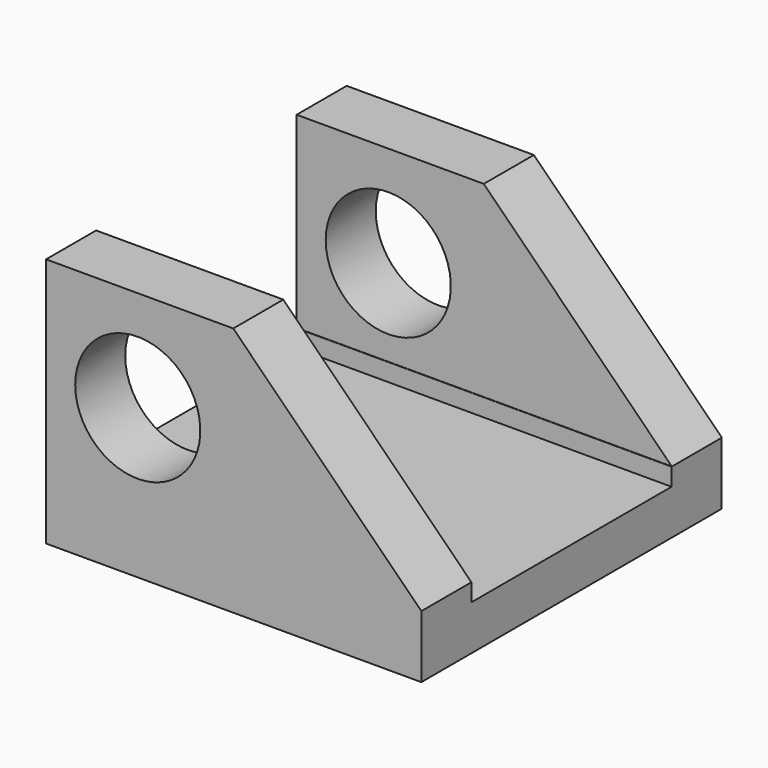
from build123d import *

# Parameters (mm, degrees)
F0_W      = 152.3780375719
F0_H      = 152.3780375719
F1_DEPTH  = 25.4
F3_W      = 76.005205512
F3_H      = 76.2
F4_DEPTH  = 25.4
F6_DEPTH  = 25.4
F9_D      = 50.8
F10_W     = 101.6018704236
F10_H     = 7.1799890138
F11_DEPTH = 152.4


with BuildPart() as f1:
    # F0 (on Top) → F1 (new body)
    with BuildSketch(Plane.XY):
        with Locations((0.1838132739, -0.0919029117)):
            Rectangle(F0_W, F0_H)
    extrude(amount=-F1_DEPTH)



with BuildPart() as f4:
    # F3 (on face) → F4 (new body)
    with BuildSketch(Plane.XZ.offset(76.2809216976)):
        with Locations((-38.002602756, 38.1)):
            Rectangle(F3_W, F3_H)
    extrude(amount=-F4_DEPTH)


with BuildPart() as f6:
    # F5 (on face) → F6 (new body)
    with BuildSketch(Plane.XZ.offset(76.2809216976)):
        Polygon((76.3728320599, 0), (0, 76.2), (0, 0), align=None)
    extrude(amount=-F6_DEPTH)


with BuildPart() as f1_1:
    add(f1.part)

    add(f4.part)  # F7 merges F4

    add(f6.part)  # F7 merges F6
    # F7: F6, F4 across plane
    add(f6.part.mirror(Plane.XZ))
    add(f4.part.mirror(Plane.XZ))

    # F9 (through all)
    with Locations(Plane.XZ.offset(76.2809216976)):
        with Locations((-38.783788681, 35.2485440671)):
            Hole(F9_D / 2)

    # F10 (on face) → F11 (cut)
    with BuildSketch(Plane.YZ.offset(76.3728320599)):
        with Locations((-0.0799864858, -3.5899945069)):
            Rectangle(F10_W, F10_H)
    extrude(amount=-F11_DEPTH, mode=Mode.SUBTRACT)


solid = f1_1.part
